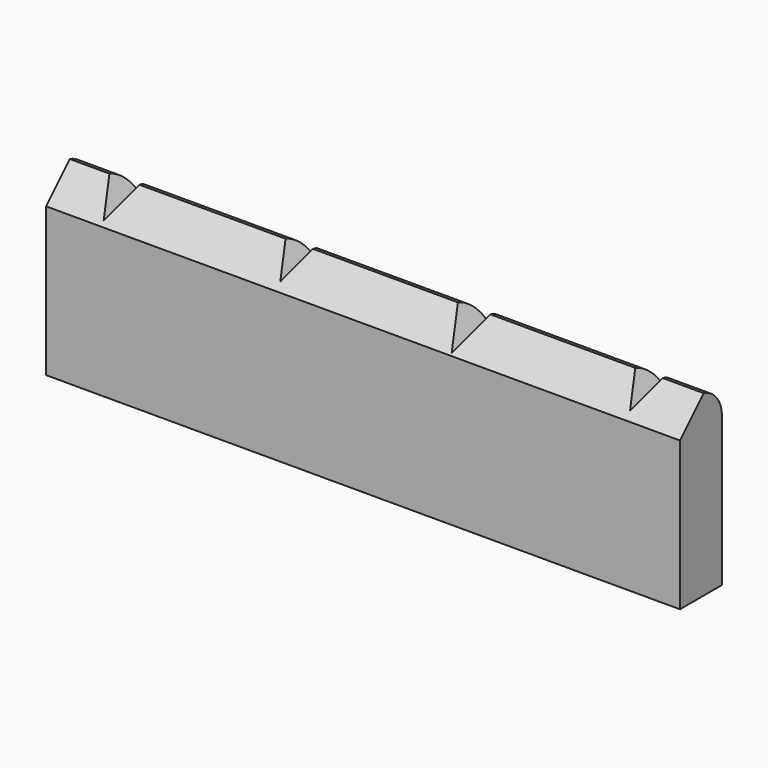
from build123d import *

# Parameters (mm, degrees)
F0_W        = 36.83
F0_H        = 3.048
F1_DEPTH    = 10.414
F3_R        = 1.778
F4_T1_DEPTH = 45.9749047052
F5_DEPTH    = 25.4


# Not quite as in the source:
# - a fillet or chamfer that OpenCascade refuses, or shapes differently, is made with other operations: its cross-section is extruded or revolved along the edge and cut away or added


with BuildPart() as f1:
    # F0 (on Top) → F1 (new body)
    with BuildSketch(Plane.XY):
        with Locations((-0.254, 1.524)):
            Rectangle(F0_W, F0_H)
    extrude(amount=F1_DEPTH)

    # F3
    f3_edges = [f1.edges().sort_by_distance(p)[0] for p in [
        (-0.254, 3.048, 10.414),
    ]]
    fillet(f3_edges, radius=F3_R)

    # F4: chamfer of 1.778 on 1 edges, made by hand

    # F4_s2 → F4_t1 (cut)
    with BuildSketch(Plane.YZ.offset(-23.2414523526)):
        Polygon((1.778, 10.414), (0, 8.636), (0, 10.414), align=None)
    extrude(amount=F4_T1_DEPTH, mode=Mode.SUBTRACT)

    # F2 (on face) → F5 (cut)
    with BuildSketch(Plane.XZ):
        Polygon((-15.494, 8.8492954744), (-14.5906174209, 10.414), (-16.3973825791, 10.414), align=None)
        Polygon((-4.5039409051, 10.414), (-6.1640590949, 10.414), (-5.334, 8.9762954744), align=None)
        Polygon((5.8027060633, 10.414), (3.8492939367, 10.414), (4.826, 8.7222954744), align=None)
        Polygon((15.8160590949, 10.414), (14.1559409051, 10.414), (14.986, 8.9762954744), align=None)
    extrude(amount=-F5_DEPTH, mode=Mode.SUBTRACT)


solid = f1.part
